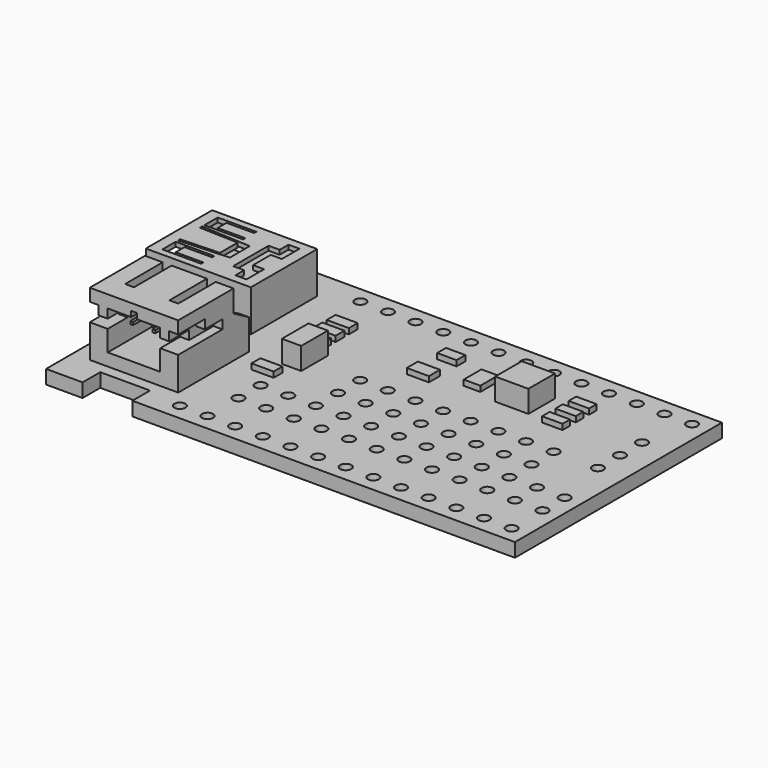
from build123d import *

# Parameters (mm, degrees)
F0_R      = 0.5
F1_DEPTH  = 1.25
F3_W      = 1.85
F3_H      = 0.85
F9_DEPTH  = 0.5
F5_W      = 1.5
F5_H      = 2
F10_DEPTH = 0.5
F6_W      = 1.75
F6_H      = 1
F11_DEPTH = 0.5
F6_W_2    = 2
F6_H_2    = 1.25
F7_W      = 2
F7_H      = 1
F12_DEPTH = 0.5
F4_W      = 3
F4_H      = 3
F13_DEPTH = 2
F8_W      = 1.75
F8_H      = 3
F14_DEPTH = 2
F16_DEPTH = 5.75
F17_W     = 9.5
F17_H     = 7.5
F18_DEPTH = 3.75
F19_W     = 4.75
F19_H     = 3.5
F20_DEPTH = 5
F22_DEPTH = 2
F24_DEPTH = 6
F26_DEPTH = 0.4
F28_DEPTH = 5
F29_W     = 0.8
F29_H     = 4.25
F30_DEPTH = 1.125
F31_W     = 0.8125
F31_H     = 0.8125
F32_DEPTH = 5
F33_DEPTH = 2.25
F34_DEPTH = 3
F36_DEPTH = 40.851
F37_W     = 0.25
F37_H     = 0.25
F38_DEPTH = 4


with BuildPart() as f1:
    # F0 (on Top) → F1 (new body)
    with BuildSketch(Plane.XY):
        Polygon((-13.4, -11.7), (21.2, -11.7), (21.2, 11.7), (-21.2, 11.7), (-21.2, -11.7), (-17.9, -11.7), (-17.9, -9.7), (-13.4, -9.7), align=None)
        with Locations((-10.3, -10.2)):
            Circle(F0_R, mode=Mode.SUBTRACT)
        with Locations((-7.8, -10.2)):
            Circle(F0_R, mode=Mode.SUBTRACT)
        with Locations((-5.3, -10.2)):
            Circle(F0_R, mode=Mode.SUBTRACT)
        with Locations((-2.8, -10.2)):
            Circle(F0_R, mode=Mode.SUBTRACT)
        with Locations((-0.3, -10.2)):
            Circle(F0_R, mode=Mode.SUBTRACT)
        with Locations((-7.8, -6.7)):
            Circle(F0_R, mode=Mode.SUBTRACT)
        with Locations((-5.3, -6.7)):
            Circle(F0_R, mode=Mode.SUBTRACT)
        with Locations((-2.8, -6.7)):
            Circle(F0_R, mode=Mode.SUBTRACT)
        with Locations((-0.3, -6.7)):
            Circle(F0_R, mode=Mode.SUBTRACT)
        with Locations((-7.8, -4.2)):
            Circle(F0_R, mode=Mode.SUBTRACT)
        with Locations((-5.3, -4.2)):
            Circle(F0_R, mode=Mode.SUBTRACT)
        with Locations((-2.8, -4.2)):
            Circle(F0_R, mode=Mode.SUBTRACT)
        with Locations((-0.3, -4.2)):
            Circle(F0_R, mode=Mode.SUBTRACT)
        with Locations((-2.8, -1.7)):
            Circle(F0_R, mode=Mode.SUBTRACT)
        with Locations((-0.3, -1.7)):
            Circle(F0_R, mode=Mode.SUBTRACT)
        with Locations((2.2, -10.2)):
            Circle(F0_R, mode=Mode.SUBTRACT)
        with Locations((4.7, -10.2)):
            Circle(F0_R, mode=Mode.SUBTRACT)
        with Locations((7.2, -10.2)):
            Circle(F0_R, mode=Mode.SUBTRACT)
        with Locations((9.7, -10.2)):
            Circle(F0_R, mode=Mode.SUBTRACT)
        with Locations((2.2, -6.7)):
            Circle(F0_R, mode=Mode.SUBTRACT)
        with Locations((4.7, -6.7)):
            Circle(F0_R, mode=Mode.SUBTRACT)
        with Locations((7.2, -6.7)):
            Circle(F0_R, mode=Mode.SUBTRACT)
        with Locations((9.7, -6.7)):
            Circle(F0_R, mode=Mode.SUBTRACT)
        with Locations((12.2, -10.2)):
            Circle(F0_R, mode=Mode.SUBTRACT)
        with Locations((14.7, -10.2)):
            Circle(F0_R, mode=Mode.SUBTRACT)
        with Locations((17.2, -10.2)):
            Circle(F0_R, mode=Mode.SUBTRACT)
        with Locations((19.7, -10.2)):
            Circle(F0_R, mode=Mode.SUBTRACT)
        with Locations((12.2, -6.7)):
            Circle(F0_R, mode=Mode.SUBTRACT)
        with Locations((14.7, -6.7)):
            Circle(F0_R, mode=Mode.SUBTRACT)
        with Locations((17.2, -6.7)):
            Circle(F0_R, mode=Mode.SUBTRACT)
        with Locations((19.7, -6.7)):
            Circle(F0_R, mode=Mode.SUBTRACT)
        with Locations((2.2, -4.2)):
            Circle(F0_R, mode=Mode.SUBTRACT)
        with Locations((4.7, -4.2)):
            Circle(F0_R, mode=Mode.SUBTRACT)
        with Locations((7.2, -4.2)):
            Circle(F0_R, mode=Mode.SUBTRACT)
        with Locations((9.7, -4.2)):
            Circle(F0_R, mode=Mode.SUBTRACT)
        with Locations((2.2, -1.7)):
            Circle(F0_R, mode=Mode.SUBTRACT)
        with Locations((4.7, -1.7)):
            Circle(F0_R, mode=Mode.SUBTRACT)
        with Locations((7.2, -1.7)):
            Circle(F0_R, mode=Mode.SUBTRACT)
        with Locations((9.7, -1.7)):
            Circle(F0_R, mode=Mode.SUBTRACT)
        with Locations((12.2, -4.2)):
            Circle(F0_R, mode=Mode.SUBTRACT)
        with Locations((14.7, -4.2)):
            Circle(F0_R, mode=Mode.SUBTRACT)
        with Locations((17.2, -4.2)):
            Circle(F0_R, mode=Mode.SUBTRACT)
        with Locations((19.7, -4.2)):
            Circle(F0_R, mode=Mode.SUBTRACT)
        with Locations((12.2, -1.7)):
            Circle(F0_R, mode=Mode.SUBTRACT)
        with Locations((14.7, -1.7)):
            Circle(F0_R, mode=Mode.SUBTRACT)
        with Locations((-2.8, 0.8)):
            Circle(F0_R, mode=Mode.SUBTRACT)
        with Locations((-0.3, 0.8)):
            Circle(F0_R, mode=Mode.SUBTRACT)
        with Locations((-10.3, 10.2)):
            Circle(F0_R, mode=Mode.SUBTRACT)
        with Locations((-7.8, 10.2)):
            Circle(F0_R, mode=Mode.SUBTRACT)
        with Locations((-5.3, 10.2)):
            Circle(F0_R, mode=Mode.SUBTRACT)
        with Locations((-2.8, 10.2)):
            Circle(F0_R, mode=Mode.SUBTRACT)
        with Locations((-0.3, 10.2)):
            Circle(F0_R, mode=Mode.SUBTRACT)
        with Locations((2.2, 0.8)):
            Circle(F0_R, mode=Mode.SUBTRACT)
        with Locations((4.7, 0.8)):
            Circle(F0_R, mode=Mode.SUBTRACT)
        with Locations((7.2, 0.8)):
            Circle(F0_R, mode=Mode.SUBTRACT)
        with Locations((9.7, 0.8)):
            Circle(F0_R, mode=Mode.SUBTRACT)
        with Locations((12.2, 0.8)):
            Circle(F0_R, mode=Mode.SUBTRACT)
        with Locations((14.7, 0.8)):
            Circle(F0_R, mode=Mode.SUBTRACT)
        with Locations((18.7, 0.8)):
            Circle(F0_R, mode=Mode.SUBTRACT)
        with Locations((18.7, 3.3)):
            Circle(F0_R, mode=Mode.SUBTRACT)
        with Locations((18.7, 5.8)):
            Circle(F0_R, mode=Mode.SUBTRACT)
        with Locations((2.2, 10.2)):
            Circle(F0_R, mode=Mode.SUBTRACT)
        with Locations((4.7, 10.2)):
            Circle(F0_R, mode=Mode.SUBTRACT)
        with Locations((7.2, 10.2)):
            Circle(F0_R, mode=Mode.SUBTRACT)
        with Locations((9.7, 10.2)):
            Circle(F0_R, mode=Mode.SUBTRACT)
        with Locations((12.2, 10.2)):
            Circle(F0_R, mode=Mode.SUBTRACT)
        with Locations((14.7, 10.2)):
            Circle(F0_R, mode=Mode.SUBTRACT)
        with Locations((17.2, 10.2)):
            Circle(F0_R, mode=Mode.SUBTRACT)
        with Locations((19.7, 10.2)):
            Circle(F0_R, mode=Mode.SUBTRACT)
    extrude(amount=F1_DEPTH)


with BuildPart() as f9:
    # F3 (on face) → F9 (new body)
    with BuildSketch(Plane.XY.offset(1.25)):
        with Locations((12.2, 4.2)):
            Rectangle(F3_W, F3_H)
    extrude(amount=F9_DEPTH)


with BuildPart() as f9b:
    # F3 (on face) → F9, piece 2 (new body)
    with BuildSketch(Plane.XY.offset(1.25)):
        with Locations((12.2, 5.7)):
            Rectangle(F3_W, F3_H)
    extrude(amount=F9_DEPTH)


with BuildPart() as f9c:
    # F3 (on face) → F9, piece 3 (new body)
    with BuildSketch(Plane.XY.offset(1.25)):
        with Locations((12.2, 7.2)):
            Rectangle(F3_W, F3_H)
    extrude(amount=F9_DEPTH)


with BuildPart() as f10:
    # F5 (on face) → F10 (new body)
    with BuildSketch(Plane.XY.offset(1.25)):
        with Locations((4.2, 5.7)):
            Rectangle(F5_W, F5_H)
    extrude(amount=F10_DEPTH)


with BuildPart() as f11:
    # F6 (on face) → F11 (new body)
    with BuildSketch(Plane.XY.offset(1.25)):
        with Locations((0.325, 7.2)):
            Rectangle(F6_W, F6_H)
    extrude(amount=F11_DEPTH)


with BuildPart() as f11b:
    # F6 (on face) → F11, piece 2 (new body)
    with BuildSketch(Plane.XY.offset(1.25)):
        with Locations((0.2, 4.2)):
            Rectangle(F6_W_2, F6_H_2)
    extrude(amount=F11_DEPTH)


with BuildPart() as f12:
    # F7 (on face) → F12 (new body)
    with BuildSketch(Plane.XY.offset(1.25)):
        with Locations((-8.8, 6.275)):
            Rectangle(F7_W, F7_H)
    extrude(amount=F12_DEPTH)


with BuildPart() as f12b:
    # F7 (on face) → F12, piece 2 (new body)
    with BuildSketch(Plane.XY.offset(1.25)):
        with Locations((-8.8, 4.775)):
            Rectangle(F7_W, F7_H)
    extrude(amount=F12_DEPTH)


with BuildPart() as f12c:
    # F7 (on face) → F12, piece 3 (new body)
    with BuildSketch(Plane.XY.offset(1.25)):
        with Locations((-8.8, 3.275)):
            Rectangle(F7_W, F7_H)
    extrude(amount=F12_DEPTH)


with BuildPart() as f12d:
    # F7 (on face) → F12, piece 4 (new body)
    with BuildSketch(Plane.XY.offset(1.25)):
        with Locations((-8.8, -2.225)):
            Rectangle(F7_W, F7_H)
    extrude(amount=F12_DEPTH)


with BuildPart() as f13:
    # F4 (on face) → F13 (new body)
    with BuildSketch(Plane.XY.offset(1.25)):
        with Locations((8.2, 5.7)):
            Rectangle(F4_W, F4_H)
    extrude(amount=F13_DEPTH)


with BuildPart() as f14:
    # F8 (on face) → F14 (new body)
    with BuildSketch(Plane.XY.offset(1.25)):
        with Locations((-7.8, 0.8)):
            Rectangle(F8_W, F8_H)
    extrude(amount=F14_DEPTH)


with BuildPart() as f16:
    # F15 (on face) → F16 (new body)
    with BuildSketch(Plane.XY.offset(1.25)):
        Polygon((-19.65, -8.7), (-11.65, -8.7), (-11.65, -0.7), (-12.45, -0.7), (-12.45, -2.45), (-18.85, -2.45), (-18.85, -0.7), (-19.65, -0.7), align=None)
    extrude(amount=F16_DEPTH)

    # F19 (on face) → F20 (cut)
    with BuildSketch(Plane.XZ.offset(8.7)):
        with Locations((-15.65, 4.125)):
            Rectangle(F19_W, F19_H)
    extrude(amount=-F20_DEPTH, mode=Mode.SUBTRACT)

    # F29 (on face) → F30 (cut, through all)
    with BuildSketch(Plane.XY.offset(7)):
        with Locations((-17.65, -4.575)):
            Rectangle(F29_W, F29_H)
        with Locations((-13.65, -4.575)):
            Rectangle(F29_W, F29_H)
    extrude(amount=-F30_DEPTH, mode=Mode.SUBTRACT)

    # F31 (on face) → F32 (cut, through all)
    with BuildSketch(Plane.XZ.offset(8.7)):
        Polygon((-15.9, 6.375), (-15.9, 5.875), (-15.4, 5.875), (-15.4, 6.375), (-15.65, 6.375), align=None)
        with Locations((-19.24375, 4.65625)):
            Rectangle(F31_W, F31_H)
        with Locations((-12.05625, 4.65625)):
            Rectangle(F31_W, F31_H)
    extrude(amount=-F32_DEPTH, mode=Mode.SUBTRACT)

    # F31 (on face) → F33 (cut)
    with BuildSketch(Plane.XZ.offset(8.7)):
        with Locations((-18.43125, 4.65625)):
            Rectangle(F31_W, F31_H)
        with Locations((-12.86875, 4.65625)):
            Rectangle(F31_W, F31_H)
    extrude(amount=-F33_DEPTH, mode=Mode.SUBTRACT)

    # F31 (on face) → F34 (cut)
    with BuildSketch(Plane.XZ.offset(8.7)):
        with Locations((-19.24375, 5.46875)):
            Rectangle(F31_W, F31_H)
        with Locations((-12.05625, 5.46875)):
            Rectangle(F31_W, F31_H)
    extrude(amount=-F34_DEPTH, mode=Mode.SUBTRACT)

    # F35 (on face) → F36 (cut, through all)
    with BuildSketch(Plane(origin=(-19.65, 0, 0), x_dir=(0, -1, 0), z_dir=(-1, 0, 0))):
        Polygon((2.45, 5), (2.45, 7), (0.7, 7), (0.7, 4), align=None)
    extrude(amount=-F36_DEPTH, mode=Mode.SUBTRACT)


with BuildPart() as f18:
    # F17 (on face) → F18 (new body)
    with BuildSketch(Plane.XY.offset(1.25)):
        with Locations((-17.95, 5.2)):
            Rectangle(F17_W, F17_H)
    extrude(amount=F18_DEPTH)

    # F21 (on face) → F22 (cut)
    with BuildSketch(Plane(origin=(-22.7, 0, 0), x_dir=(0, -1, 0), z_dir=(-1, 0, 0))):
        Polygon((-8.95, 1.25), (-8.45, 1.25), (-8.45, 2.625), (-8.95, 3.125), align=None)
        Polygon((-1.95, 2.625), (-1.95, 1.25), (-1.45, 1.25), (-1.45, 3.125), align=None)
    extrude(amount=-F22_DEPTH, mode=Mode.SUBTRACT)

    # F23 (on face) → F24 (cut)
    with BuildSketch(Plane(origin=(-22.7, 0, 0), x_dir=(0, -1, 0), z_dir=(-1, 0, 0))):
        Polygon((-1.85, 4.6), (-8.55, 4.6), (-8.55, 3.3688763524), (-8.05, 2.625), (-8.05, 1.65), (-2.35, 1.65), (-2.35, 2.625), (-1.85, 3.3688763524), align=None)
    extrude(amount=-F24_DEPTH, mode=Mode.SUBTRACT)

    # F25 (on face) → F26 (cut, through all)
    with BuildSketch(Plane.XY.offset(5)):
        Polygon((-17.2, 4.075), (-17.2, 5.2), (-17.2, 6.325), (-21.7, 6.575), (-21.7, 6.325), (-18.2, 6.2), (-18.2, 5.2), (-18.2, 4.2), (-21.7, 4.075), (-21.7, 3.825), align=None)
        Polygon((-18.2, 8.075), (-18.2, 8.325), (-21.7, 8.325), (-21.7, 6.825), (-18.2, 6.825), (-18.2, 7.075), (-20.7, 7.075), (-20.7, 8.075), align=None)
        Polygon((-14.2, 6.2), (-14.2, 8.2), (-15.2, 8.2), (-15.2, 7.2), (-16.2, 7.2), (-16.2, 5.2), (-16.2, 3.2), (-15.2, 3.2), (-15.2, 2.2), (-14.2, 2.2), (-14.2, 4.2), (-15.2, 4.2), (-15.2, 5.2), (-15.2, 6.2), align=None)
        Polygon((-18.2, 2.075), (-18.2, 2.325), (-20.7, 2.325), (-20.7, 3.325), (-18.2, 3.325), (-18.2, 3.575), (-21.7, 3.575), (-21.7, 2.075), align=None)
    extrude(amount=-F26_DEPTH, mode=Mode.SUBTRACT)


with BuildPart() as f28:
    # F27 (on face) → F28 (new body)
    with BuildSketch(Plane(origin=(-16.7, 0, 0), x_dir=(0, -1, 0), z_dir=(-1, 0, 0))):
        Polygon((-2.825, 3.4), (-7.575, 3.4), (-7.575, 2.65), (-6.575, 1.9), (-3.825, 1.9), (-2.825, 2.65), align=None)
    extrude(amount=F28_DEPTH)


with BuildPart() as f38:
    # F37 (on face) → F38 (new body)
    with BuildSketch(Plane.XZ.offset(3.7)):
        with Locations((-16.65, 4.75)):
            Rectangle(F37_W, F37_H)
    extrude(amount=F38_DEPTH)


with BuildPart() as f38b:
    # F37 (on face) → F38, piece 2 (new body)
    with BuildSketch(Plane.XZ.offset(3.7)):
        with Locations((-14.65, 4.75)):
            Rectangle(F37_W, F37_H)
    extrude(amount=F38_DEPTH)


solid = Compound([f1.part, f9.part, f9b.part, f9c.part, f10.part, f11.part, f11b.part, f12.part, f12b.part, f12c.part, f12d.part, f13.part, f14.part, f16.part, f18.part, f28.part, f38.part, f38b.part])
